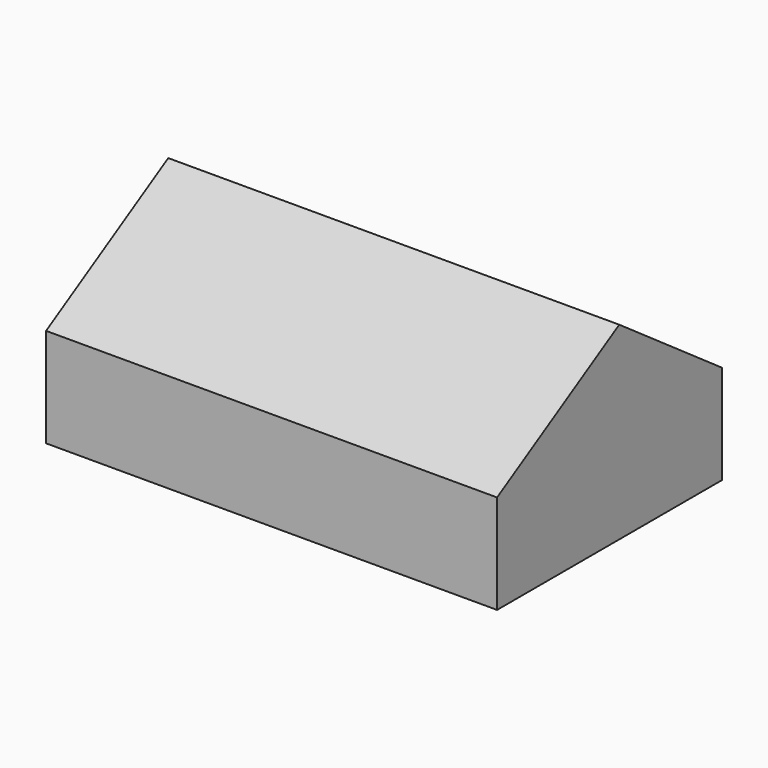
from build123d import *

# Parameters (mm, degrees)
F0_R      = 0.6477
F0_R_2    = 0.6441405576
F1_DEPTH  = 25.4
F2_W      = 127.2426065671
F2_H      = 43.082173756
F3_DEPTH  = 25.4
F6_DEPTH  = 127.2436065671
F7_W      = 127.2426065671
F7_H      = 36.2138515522
F8_DEPTH  = 25.4
F11_DEPTH = 127.2436065671
F12_W     = 127.2426065671
F12_H     = 79.2960253082
F13_DEPTH = 2.54


# Not quite as in the source:
# - ends of sketch curves that miss each other by under 0.0002 mm in the source are joined


with BuildPart() as f1:
    # F0 (on Top) → F1 (new body)
    with BuildSketch(Plane.XY):
        Polygon((-47.2229928794, 27.8801387091), (-47.2229928794, 30.4201387091), (-44.6829928794, 30.4201387091), (2.3896338216, 30.4201387091), (2.3896338216, 33.6738515522), (2.3896338216, 36.2138515522), (-62.2987892685, 36.2138515522), (-62.2987892685, 19.4619052569), (-59.7587892685, 19.4619052569), (-47.2229928794, 19.4619052569), align=None)
        Polygon((-44.6829928794, 30.4201387091), (-47.2229928794, 30.4201387091), (-47.2229928794, 27.8801387091), (-47.2229928794, 19.4619052569), (-59.7587892685, 19.4619052569), (-62.2987892685, 19.4619052569), (-62.2987892685, 16.9219052569), (-62.2987892685, -29.6174437481), (-62.2987892685, -32.1574437481), (-59.7587892685, -32.1574437481), (-16.2234111885, -32.1574437481), (-13.6834111885, -32.1574437481), (-13.6834111885, -29.6174437481), (-13.6834111885, -19.4574437481), (9.1386072609, -19.4574437481), (9.1386072609, -40.542173756), (9.1386072609, -43.082173756), (11.6786072609, -43.082173756), (32.1430532363, -43.082173756), (34.6830532363, -43.082173756), (34.6830532363, -40.542173756), (34.6830532363, -19.4574437481), (62.4038172987, -19.4574437481), (62.4038172987, -16.9174437481), (34.6830532363, -16.9174437481), (32.1430532363, -16.9174437481), (32.1430532363, -19.4574437481), (32.1430532363, -40.542173756), (11.6786072609, -40.542173756), (11.6786072609, -19.4574437481), (11.6786072609, -16.9174437481), (9.1386072609, -16.9174437481), (-13.6834111885, -16.9174437481), (-16.2234111885, -16.9174437481), (-16.2234111885, -19.4574437481), (-16.2234111885, -29.6174437481), (-59.7587892685, -29.6174437481), (-59.7587892685, 1.3920115222), (-59.7587892685, 2.6620115222), (-59.7587892685, 16.9219052569), (-47.2229928794, 16.9219052569), (-45.9529928794, 16.9219052569), (-44.6829928794, 16.9219052569), (-44.6829928794, 19.4619052569), (-44.6829928794, 27.8801387091), (2.3896338216, 27.8801387091), (4.9296338216, 27.8801387091), (4.9296338216, 30.4201387091), (4.9296338216, 33.6738515522), (11.6786072609, 33.6738515522), (11.6786072609, 30.4201387091), (11.6786072609, 27.8801387091), (14.2186072609, 27.8801387091), (62.4038172987, 27.8801387091), (62.4038172987, 30.4201387091), (14.2186072609, 30.4201387091), (14.2186072609, 33.6738515522), (14.2186072609, 36.2138515522), (11.6786072609, 36.2138515522), (4.9296338216, 36.2138515522), (2.3896338216, 36.2138515522), (2.3896338216, 33.6738515522), (2.3896338216, 30.4201387091), align=None)
        with Locations((-61.0287892685, -30.8874437481)):
            Circle(F0_R, mode=Mode.SUBTRACT)
        with Locations((-14.9534111885, -30.8874437481)):
            Circle(F0_R, mode=Mode.SUBTRACT)
        with Locations((-14.9534111885, -18.1874437481)):
            Circle(F0_R, mode=Mode.SUBTRACT)
        with Locations((10.4086072609, -41.812173756)):
            Circle(F0_R, mode=Mode.SUBTRACT)
        with Locations((33.4130532363, -41.812173756)):
            Circle(F0_R, mode=Mode.SUBTRACT)
        with Locations((10.4086072609, -18.1874437481)):
            Circle(F0_R, mode=Mode.SUBTRACT)
        with Locations((33.4130532363, -18.1874437481)):
            Circle(F0_R, mode=Mode.SUBTRACT)
        with Locations((-61.0287892685, 18.1919052569)):
            Circle(F0_R, mode=Mode.SUBTRACT)
        with Locations((-45.9529928794, 18.1919052569)):
            Circle(F0_R, mode=Mode.SUBTRACT)
        with Locations((-45.9529928794, 29.1501387091)):
            Circle(F0_R_2, mode=Mode.SUBTRACT)
        with Locations((3.6596338216, 29.1501387091)):
            Circle(F0_R, mode=Mode.SUBTRACT)
        with Locations((12.9486072609, 29.1501387091)):
            Circle(F0_R, mode=Mode.SUBTRACT)
        with Locations((3.6596338216, 34.9438515522)):
            Circle(F0_R, mode=Mode.SUBTRACT)
        with Locations((12.9486072609, 34.9438515522)):
            Circle(F0_R, mode=Mode.SUBTRACT)
        Polygon((64.9438172987, 36.2138515522), (14.2186072609, 36.2138515522), (14.2186072609, 33.6738515522), (14.2186072609, 30.4201387091), (62.4038172987, 30.4201387091), (64.9438172987, 30.4201387091), align=None)
        Polygon((-59.7587892685, -32.1574437481), (-62.2987892685, -32.1574437481), (-62.2987892685, -43.082173756), (9.1386072609, -43.082173756), (9.1386072609, -40.542173756), (9.1386072609, -19.4574437481), (-13.6834111885, -19.4574437481), (-13.6834111885, -29.6174437481), (-13.6834111885, -32.1574437481), (-16.2234111885, -32.1574437481), align=None)
        Polygon((64.9438172987, 27.8801387091), (64.9438172987, 30.4201387091), (62.4038172987, 30.4201387091), (62.4038172987, 27.8801387091), (62.4038172987, 2.6620115222), (62.4038172987, 1.3920115222), (62.4038172987, -16.9174437481), (62.4038172987, -19.4574437481), (64.9438172987, -19.4574437481), (64.9438172987, -16.9174437481), align=None)
        with Locations((63.6738172987, -18.1874437481)):
            Circle(F0_R, mode=Mode.SUBTRACT)
        with Locations((63.6738172987, 29.1501387091)):
            Circle(F0_R, mode=Mode.SUBTRACT)
        Polygon((64.9438172987, -43.082173756), (64.9438172987, -19.4574437481), (62.4038172987, -19.4574437481), (34.6830532363, -19.4574437481), (34.6830532363, -40.542173756), (34.6830532363, -43.082173756), align=None)
    extrude(amount=F1_DEPTH)

    # F2 (on face) → F3 (join)
    with BuildSketch(Plane.XY.offset(25.4)):
        with Locations((1.3225140151, -21.541086878)):
            Rectangle(F2_W, F2_H)
    extrude(amount=F3_DEPTH)

    # F5 (on face) → F6 (cut, through all)
    with BuildSketch(Plane.YZ.offset(64.9438172987)):
        Polygon((-43.082173756, 50.8), (-43.082173756, 25.4001487046), (0, 50.7993288338), (0, 50.8), align=None)
    extrude(amount=-F6_DEPTH, mode=Mode.SUBTRACT)

    # F7 (on face) → F8 (join)
    with BuildSketch(Plane.XY.offset(25.4)):
        with Locations((1.3225140151, 18.1069257761)):
            Rectangle(F7_W, F7_H)
    extrude(amount=F8_DEPTH)

    # F9 (on face) → F11 (cut, through all)
    with BuildSketch(Plane(origin=(-62.2987892685, 0, 0), x_dir=(0, -1, 0), z_dir=(-1, 0, 0))):
        Polygon((-36.2138515522, 25.4), (0, 50.7996644169), (0, 50.8), (-36.2138515522, 50.8), align=None)
    extrude(amount=-F11_DEPTH, mode=Mode.SUBTRACT)

    # F12 (on face) → F13 (join)
    with BuildSketch(Plane(origin=(0, 0, 0), x_dir=(1, 0, 0), z_dir=(0, 0, -1))):
        with Locations((1.3225140151, 3.4341611019)):
            Rectangle(F12_W, F12_H)
    extrude(amount=F13_DEPTH)


solid = f1.part
